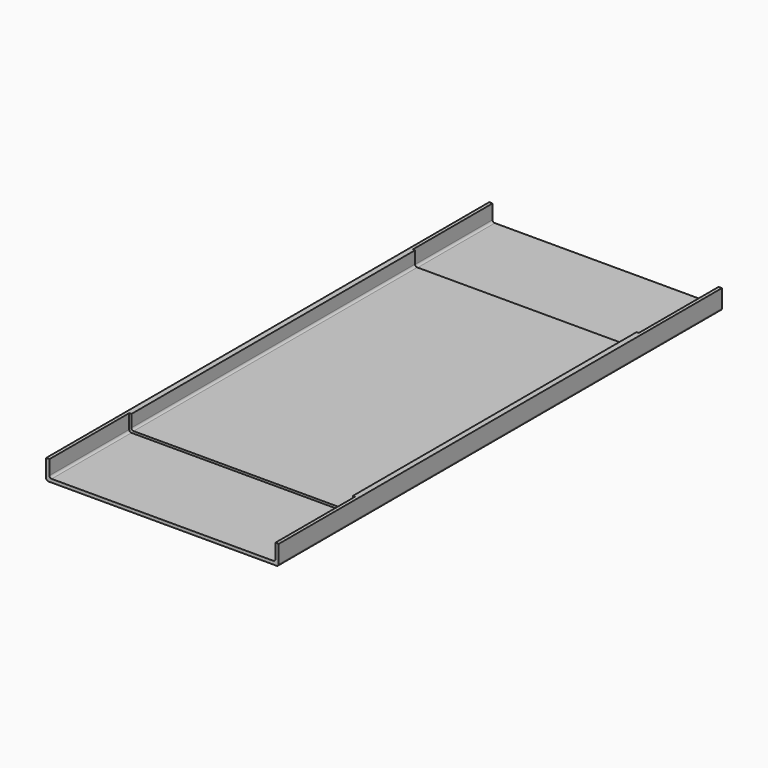
from build123d import *

# Parameters (mm, degrees)
F1_DEPTH = 500
F2_DEPTH = 90


# Not quite as in the source:
# - a pattern or mirror of a feature is missing from the dataset's text; its kind, count and spacing are read off the source's solid


with BuildPart() as f1:
    # F0 (on Front) → F1 (new body)
    with BuildSketch(Plane.XZ):
        with BuildLine():
            Line((102, 0), (100, 0))
            Line((100, 0), (100, -11))
            ThreePointArc((100, -11), (99.4142135624, -12.4142135624), (98, -13))
            Line((98, -13), (0, -13))
            Line((0, -13), (-98, -13))
            ThreePointArc((-98, -13), (-99.4142135624, -12.4142135624), (-100, -11))
            Line((-100, -11), (-100, 0))
            Line((-100, 0), (-102, 0))
            Line((-102, 0), (-102, -13))
            ThreePointArc((-102, -13), (-101.4142135624, -14.4142135624), (-100, -15))
            Line((-100, -15), (100, -15))
            ThreePointArc((100, -15), (101.4142135624, -14.4142135624), (102, -13))
            Line((102, -13), (102, 0))
        make_face()
        with BuildLine():
            Line((105, 0), (102, 0))
            Line((102, 0), (102, -13))
            ThreePointArc((102, -13), (101.4142135624, -14.4142135624), (100, -15))
            Line((100, -15), (-100, -15))
            ThreePointArc((-100, -15), (-101.4142135624, -14.4142135624), (-102, -13))
            Line((-102, -13), (-102, 0))
            Line((-102, 0), (-105, 0))
            Line((-105, 0), (-105, -16))
            ThreePointArc((-105, -16), (-104.4142135624, -17.4142135624), (-103, -18))
            Line((-103, -18), (0, -18))
            Line((0, -18), (103, -18))
            ThreePointArc((103, -18), (104.4142135624, -17.4142135624), (105, -16))
            Line((105, -16), (105, 0))
        make_face()
    extrude(amount=F1_DEPTH)

    # F0 (on Front) → F2 (cut)
    with BuildSketch(Plane.XZ):
        with BuildLine():
            Line((102, 0), (100, 0))
            Line((100, 0), (100, -11))
            ThreePointArc((100, -11), (99.4142135624, -12.4142135624), (98, -13))
            Line((98, -13), (0, -13))
            Line((0, -13), (-98, -13))
            ThreePointArc((-98, -13), (-99.4142135624, -12.4142135624), (-100, -11))
            Line((-100, -11), (-100, 0))
            Line((-100, 0), (-102, 0))
            Line((-102, 0), (-102, -13))
            ThreePointArc((-102, -13), (-101.4142135624, -14.4142135624), (-100, -15))
            Line((-100, -15), (100, -15))
            ThreePointArc((100, -15), (101.4142135624, -14.4142135624), (102, -13))
            Line((102, -13), (102, 0))
        make_face()
    f2 = extrude(amount=F2_DEPTH, mode=Mode.SUBTRACT)

    # F2_copies: F2 across plane
    add(f2.mirror(Plane(origin=(0, -250, 0), x_dir=(0, 0, -1), z_dir=(0, -1, 0))), mode=Mode.SUBTRACT)


solid = f1.part
